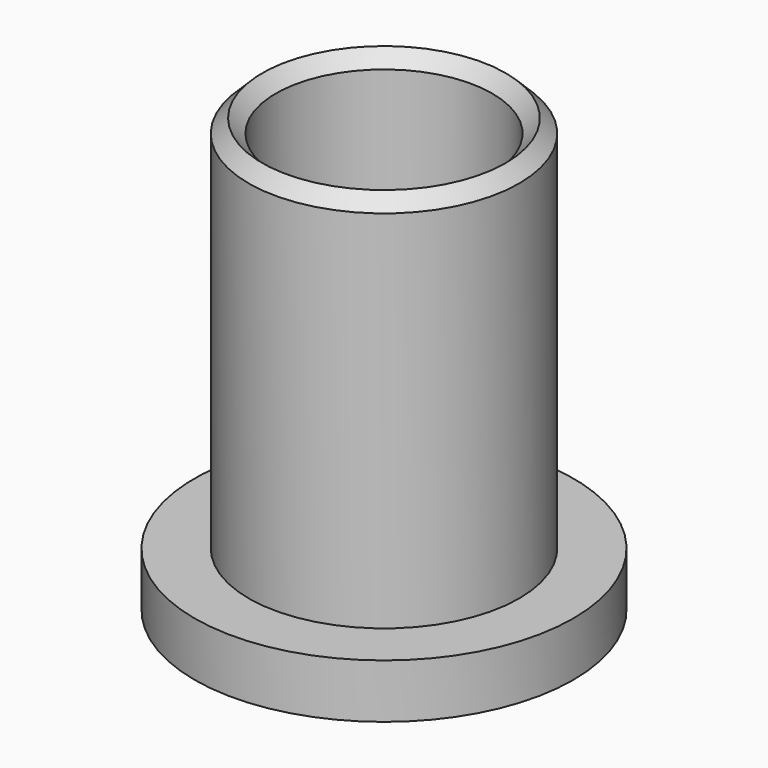
from build123d import *

# Parameters (mm, degrees)
F0_R     = 7
F1_DEPTH = 2
F2_R     = 5
F2_R_2   = 4
F3_DEPTH = 14
F4_SIZE  = 0.49999


# Not quite as in the source:
# - a fillet or chamfer is up to 0.001 mm smaller than in the source, because OpenCascade refuses the exact size


with BuildPart() as f1:
    # F0 (on Top) → F1 (new body)
    with BuildSketch(Plane.XY):
        Circle(F0_R)
    extrude(amount=F1_DEPTH)

    # F2 (on face) → F3 (join)
    with BuildSketch(Plane.XY.offset(2)):
        Circle(F2_R)
        Circle(F2_R_2, mode=Mode.SUBTRACT)
    extrude(amount=F3_DEPTH)

    # F4 (size 0.5 in the source; OpenCascade refuses exactly that, so slightly less here)
    f4_edges = [f1.edges().sort_by_distance(p)[0] for p in [
        (-5, 0, 16),
        (-4, 0, 16),
    ]]
    chamfer(f4_edges, length=F4_SIZE)


solid = f1.part
